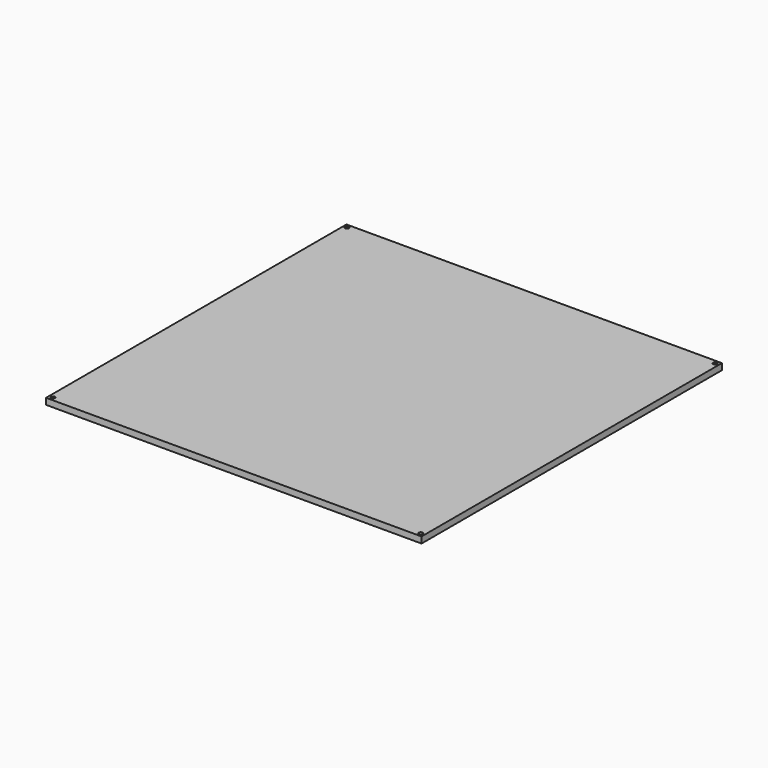
from build123d import *

# Parameters (mm, degrees)
F0_W     = 300
F0_H     = 300
F1_DEPTH = 5
F3_D     = 3.2


with BuildPart() as f1:
    # F0 (on Top) → F1 (new body)
    with BuildSketch(Plane.XY):
        with Locations((165, -165)):
            Rectangle(F0_W, F0_H)
    extrude(amount=F1_DEPTH)

    # F3 (through all)
    with Locations(Plane.XY.offset(5)):
        with Locations((18, -18), (312, -18), (312, -312), (18, -312)):
            Hole(F3_D / 2)


solid = f1.part
